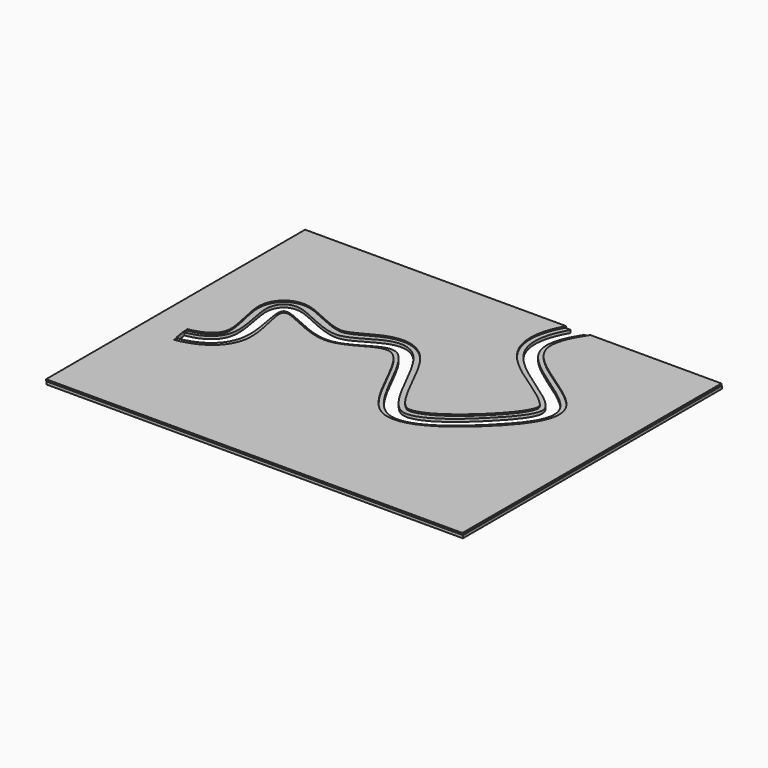
from build123d import *

# Parameters (mm, degrees)
F0_W          = 900
F0_H          = 700
F2_DEPTH      = 3
F3_DEPTH      = 25
F3_DEPTH_BACK = 25
F6_DEPTH      = 25
F6_DEPTH_BACK = 25
F7_W          = 900
F7_H          = 700
F9_DEPTH      = 6


# Not quite as in the source:
# - the dataset's text gives a spline's control points without its knots; the knots are read off the source's solid


with BuildPart() as f2:
    # F0 (on Top) → F2 (new body)
    with BuildSketch(Plane.XY):
        with Locations((136.779838565, 140.37967287)):
            Rectangle(F0_W, F0_H)
    extrude(amount=F2_DEPTH)

    # F1 (on Top) → F3 (cut, two sides)
    with BuildSketch(Plane.XY) as f3_sk:
        with BuildLine():
            Line((-241.4856788522, 82.2124957097), (-234.3062907457, 37.7888940275))
            add(Edge.make_bspline(
                [(-234.3062907457, 37.7888940275), (-183.2200698821, 46.0450414938), (-107.8197896412, 102.2279372719), (-192.2750551174, 283.579620296), (-24.0171318012, 149.9224145171), (99.4434854713, 307.8000943084), (175.8744786158, -38.137750164), (392.3120352571, 121.8215640239), (495.7588052716, 272.9639793915), (212.09229922, 380.1642280608), (301.8253737576, 491.1332534511), (345.4286754131, 545.0569987297)],
                knots=[0, 0, 0, 0, 0.1005186811, 0.1948714664, 0.2944457767, 0.3919205483, 0.524446972, 0.6500546131, 0.7560619639, 0.8852543369, 1, 1, 1, 1], degree=3))
            Line((345.4286754131, 545.0569987297), (310.4370311075, 573.3516064985))
            add(Edge.make_bspline(
                [(-241.4856788522, 82.2124957097), (-235.5376995244, 83.1737606775), (-227.1834080935, 85.1443072797), (-217.474364878, 88.6042185531), (-210.9663273096, 91.5416769635), (-205.2747075425, 94.7414795634), (-200.4160544418, 98.1187472011), (-196.373293023, 101.5953254918), (-193.0908775239, 105.1164927775), (-190.4790946185, 108.673215132), (-188.772395717, 111.7142206402), (-187.6443639611, 114.2600259837), (-186.91078749, 116.2492961693), (-186.2869465038, 118.3436017222), (-185.8604232074, 120.1988345417), (-185.5789375302, 121.7627021332), (-185.3991590865, 122.9783217928), (-185.252302169, 124.2414938638), (-185.1405994233, 125.5490498855), (-185.059563113, 126.9970714119), (-185.0000994287, 129.0879426638), (-185.0248632154, 131.9899533939), (-185.2286698235, 135.8675595467), (-185.6086882806, 140.0794825573), (-186.1581698074, 144.5682595729), (-187.0987121971, 150.8533570489), (-188.6205679067, 159.1522141918), (-190.8240279465, 169.5043124094), (-192.8083784067, 178.2695336381), (-194.3818406654, 185.3095616522), (-195.5285456157, 190.6070149505), (-196.6143456264, 195.9387036323), (-197.6084875244, 201.3452092887), (-198.4727294543, 206.9018156809), (-199.1496740668, 212.7389962035), (-199.4764712019, 218.0162233827), (-199.4894720296, 222.6632212336), (-199.3258979633, 226.4234804566), (-198.919614654, 230.5290516319), (-198.1659289654, 235.0572516522), (-196.9118918995, 240.0783575162), (-194.9451306123, 245.6253274688), (-192.4879995558, 250.6392221678), (-189.898614037, 254.7703034363), (-187.6218228143, 257.8777610524), (-184.9992992364, 260.934338153), (-182.0377655849, 263.8704376875), (-179.3129029064, 266.1548327791), (-177.000331504, 267.8542399638), (-174.6237907367, 269.4492377395), (-171.6062006951, 271.2068826251), (-167.9761634622, 272.9460428746), (-164.409661789, 274.3311498765), (-159.8065692755, 275.749902793), (-154.4349269126, 276.8203829827), (-148.7149350442, 277.3109893938), (-143.6791934777, 277.2781780434), (-139.2282351443, 276.9098327801), (-135.2505889333, 276.3274056454), (-131.6452560188, 275.6060761092), (-128.327829438, 274.7915830848), (-124.1994201874, 273.6177648935), (-119.454378243, 272.0297965106), (-114.1330202601, 269.9985841874), (-109.0163936944, 267.8708559657), (-104.0042481448, 265.6683344255), (-99.0398525291, 263.4119036969), (-94.0934068391, 261.1245526128), (-87.5071738324, 258.0675515109), (-79.2894636179, 254.301217329), (-69.5603592504, 250.1084557216), (-61.7384184503, 247.0939974118), (-55.7995425295, 245.0842808334), (-51.5499774528, 243.8013204219), (-47.5536122712, 242.7614646682), (-43.8633351999, 241.9756441117), (-41.0890345702, 241.5330763696), (-39.0767461943, 241.2996839349), (-37.6771518248, 241.1816399507), (-36.3922517161, 241.116479596), (-35.4214542607, 241.1018193712), (-34.7043651988, 241.1108325263), (-34.2011207672, 241.1268350515), (-33.6853437819, 241.1532206705), (-32.9848262391, 241.2026104861), (-32.080215541, 241.2918119898), (-30.9425191435, 241.4457711216), (-29.747492374, 241.6498724502), (-28.0732155104, 241.9930222828), (-25.822720168, 242.5627626208), (-21.880330047, 243.7981397699), (-16.331982542, 245.9761062402), (-8.8118359212, 249.5607949136), (-0.5434559099, 253.9526763782), (8.4508129905, 258.9262639267), (16.6403545663, 263.3417972682), (23.7599841554, 266.8841366803), (29.4467345634, 269.4962211057), (35.5566372376, 272.0010306462), (42.1823374373, 274.311405811), (49.4236395705, 276.3023826176), (57.3672041666, 277.795696083), (66.0465099256, 278.5509411968), (75.3837631228, 278.2821676865), (83.5113265637, 276.9778692101), (89.2081655274, 275.4330144664), (92.4367063904, 274.3708027239), (94.8382851466, 273.4852798104), (96.8161375588, 272.6754654295), (98.3841938016, 271.9843530185), (99.9262943401, 271.2721286966), (101.8038878917, 270.3453559302), (104.702705147, 268.7934917732), (108.1317869173, 266.7405344791), (111.9541425106, 264.1395026786), (115.5087239258, 261.4346763787), (119.927069824, 257.7228957042), (124.9169432693, 252.9328275462), (130.2508034542, 247.026543135), (135.0896327978, 240.9927455699), (139.554556696, 234.8416200953), (145.1283850319, 226.4875741975), (151.5589218926, 215.7632245239), (158.7710272688, 202.497891756), (165.6801971146, 188.9538806141), (172.4151365402, 175.2994869993), (179.0582911899, 161.7422451206), (185.660525585, 148.5206349377), (192.2444338178, 135.8994918833), (198.8008182512, 124.1678836236), (205.2768380346, 113.6369815809), (210.5101981, 106.1358052224), (214.4899104198, 101.0609993718), (217.3303617383, 97.7534217065), (219.978464374, 94.9733838681), (222.3765020584, 92.7378899598), (224.1137016073, 91.3274700325), (225.3142899389, 90.4567825785), (226.1163341361, 89.924057213), (226.8029845386, 89.5091405515), (227.4733439715, 89.1430138534), (228.1291176651, 88.822150909), (228.9996846256, 88.4432304879), (230.1054945245, 88.0467609434), (231.54537094, 87.6664964427), (233.1753732843, 87.3794091452), (235.057273097, 87.2021281247), (237.2335796296, 87.1635396823), (240.55731177, 87.3413929062), (245.5227987888, 88.079008451), (252.6791739242, 89.9923664451), (260.8301872351, 93.0264381942), (269.7570797741, 97.1825815618), (279.2556215065, 102.4009159936), (289.1468102787, 108.584934908), (299.2760739512, 115.6176345184), (309.5093899796, 123.3712014191), (319.7287874812, 131.7124258746), (329.8286859902, 140.5058445218), (338.0648038503, 148.0964177817), (344.5013770548, 154.2589683131), (348.4500767297, 158.1321041895), (351.5636214838, 161.2392515861), (354.6286384304, 164.3330415235), (358.3546871655, 168.163507658), (362.6480774345, 172.6981225537), (368.1173165148, 178.6510472941), (374.4439024175, 185.8985119346), (381.1201011492, 194.2088317575), (386.7882817119, 202.0338405705), (391.3723846707, 209.2487053252), (394.8283570488, 215.7004013288), (397.1689795838, 221.2164346332), (398.274140703, 224.8961691748), (398.7586304729, 227.2523477751), (398.9589780282, 228.7346603805), (399.033607176, 229.9543070221), (399.0177225056, 230.952451348), (398.9374713249, 231.7885688151), (398.8035372952, 232.5375385066), (398.6059933192, 233.282855915), (398.3615456687, 233.9702274749), (398.0917291127, 234.596295897), (397.885446547, 235.0253148368), (397.6933380765, 235.3947640399), (397.5351601954, 235.6845823574), (397.3594254936, 235.9919532357), (397.0874783947, 236.4470374628), (396.679784191, 237.0891477727), (395.8733663132, 238.2656919148), (394.567493912, 239.9926785021), (392.5131211223, 242.4074256407), (389.137265676, 246.0021498199), (383.7741089396, 251.0640022626), (375.751488869, 257.7405013236), (366.417496646, 264.8362812315), (356.0404038889, 272.2467658517), (344.8731898776, 279.9209527707), (333.1509121216, 287.8448474083), (321.0910339513, 296.0335168672), (308.893794176, 304.5289467569), (296.7425913103, 313.4033633299), (284.8049272706, 322.7684284522), (273.237915057, 332.7926592747), (264.0409228143, 341.9040126463), (257.0563649981, 349.8326975335), (252.0449681123, 356.1585682546), (248.1020472958, 361.7995109897), (245.1253394442, 366.5665889108), (242.9935925432, 370.2770521418), (241.3129881952, 373.4859400827), (240.0325980452, 376.1290050305), (238.8113517142, 378.7924683854), (237.3946194858, 382.1615894078), (235.3686208631, 387.6220814248), (233.2949562773, 394.552809555), (231.546773022, 402.9453959487), (230.5193972595, 411.3225036077), (230.1719914596, 419.6044271535), (230.4480888242, 427.7291455333), (231.5621988176, 438.2982923287), (234.1862414869, 450.9526422368), (238.8303853448, 465.2427656184), (244.6130062197, 478.7677873011), (251.2809191489, 491.6831883403), (258.6500420567, 504.1296805595), (266.5761934981, 516.2184522105), (274.935846315, 528.0312592745), (283.6149215817, 539.6249662726), (295.464949001, 554.8390039644), (304.4995700078, 566.0088107058), (310.4370311075, 573.3516064985)],
                knots=[0, 0, 0, 0, 0.015625, 0.0234375, 0.03125, 0.0390625, 0.046875, 0.0546875, 0.0625, 0.0703125, 0.078125, 0.08203125, 0.0859375, 0.08984375, 0.09375, 0.095703125, 0.09765625, 0.099609375, 0.1015625, 0.103515625, 0.10546875, 0.109375, 0.11328125, 0.1171875, 0.12109375, 0.125, 0.1328125, 0.140625, 0.1484375, 0.15234375, 0.15625, 0.16015625, 0.1640625, 0.16796875, 0.171875, 0.17578125, 0.177734375, 0.1796875, 0.181640625, 0.18359375, 0.185546875, 0.1875, 0.189453125, 0.1904296875, 0.19140625, 0.1923828125, 0.193359375, 0.1943359375, 0.1948242188, 0.1953125, 0.1962890625, 0.197265625, 0.1982421875, 0.19921875, 0.201171875, 0.203125, 0.205078125, 0.20703125, 0.208984375, 0.2109375, 0.212890625, 0.21484375, 0.21875, 0.22265625, 0.2265625, 0.23046875, 0.234375, 0.23828125, 0.2421875, 0.25, 0.2578125, 0.265625, 0.26953125, 0.2734375, 0.27734375, 0.28125, 0.28515625, 0.287109375, 0.2890625, 0.291015625, 0.29296875, 0.2939453125, 0.294921875, 0.2958984375, 0.296875, 0.298828125, 0.30078125, 0.302734375, 0.3046875, 0.30859375, 0.3125, 0.3203125, 0.328125, 0.3359375, 0.34375, 0.3515625, 0.35546875, 0.359375, 0.36328125, 0.3671875, 0.37109375, 0.375, 0.37890625, 0.3828125, 0.38671875, 0.388671875, 0.3896484375, 0.390625, 0.3916015625, 0.3920898438, 0.392578125, 0.3935546875, 0.39453125, 0.396484375, 0.3984375, 0.400390625, 0.40234375, 0.40625, 0.41015625, 0.4140625, 0.41796875, 0.421875, 0.4296875, 0.4375, 0.4453125, 0.453125, 0.4609375, 0.46875, 0.4765625, 0.484375, 0.4921875, 0.5, 0.50390625, 0.5078125, 0.51171875, 0.515625, 0.51953125, 0.521484375, 0.5234375, 0.525390625, 0.52734375, 0.529296875, 0.53125, 0.53515625, 0.5390625, 0.54296875, 0.546875, 0.55078125, 0.5546875, 0.5625, 0.5703125, 0.578125, 0.5859375, 0.59375, 0.6015625, 0.609375, 0.6171875, 0.625, 0.6328125, 0.640625, 0.64453125, 0.6484375, 0.650390625, 0.65234375, 0.65625, 0.66015625, 0.6640625, 0.671875, 0.6796875, 0.6875, 0.6953125, 0.703125, 0.7109375, 0.71875, 0.72265625, 0.7265625, 0.73046875, 0.734375, 0.73828125, 0.7421875, 0.74609375, 0.75, 0.751953125, 0.75390625, 0.7548828125, 0.755859375, 0.7568359375, 0.7578125, 0.759765625, 0.76171875, 0.765625, 0.76953125, 0.7734375, 0.78125, 0.7890625, 0.796875, 0.8046875, 0.8125, 0.8203125, 0.828125, 0.8359375, 0.84375, 0.8515625, 0.859375, 0.8671875, 0.87109375, 0.875, 0.87890625, 0.880859375, 0.8828125, 0.884765625, 0.8857421875, 0.88671875, 0.888671875, 0.890625, 0.89453125, 0.8984375, 0.90234375, 0.90625, 0.91015625, 0.9140625, 0.921875, 0.9296875, 0.9375, 0.9453125, 0.953125, 0.9609375, 0.96875, 0.9765625, 0.984375, 1, 1, 1, 1], degree=3))
        make_face()
    extrude(amount=F3_DEPTH, mode=Mode.SUBTRACT)
    extrude(f3_sk.sketch, amount=-F3_DEPTH_BACK, mode=Mode.SUBTRACT)


with BuildPart() as f2_1:
    # F5: moved
    add(f2.part.moved(Location((-139, -139, 6))))


with BuildPart() as f6:
    # F4 (on Top) → F6 (new body, two sides)
    with BuildSketch(Plane.XY) as f6_sk:
        with BuildLine():
            Line((-333.2689129169, -208.5999996712), (-329.2803639689, -233.2797783835))
            add(Edge.make_bspline(
                [(-329.2803639689, -233.2797783835), (-279.6440862088, -225.2579591544), (-215.0591975226, -169.0019007955), (-290.3221170229, 10.7279443108), (-115.933229477, -128.5278182105), (8.6171027688, 40.169951089), (91.4360122328, -317.6582258257), (294.4798541771, -146.0859910696), (390.4461045585, -16.0719332642), (105.2391975094, 95.5185231878), (204.8334747082, 217.5691570301), (250.45460219, 273.9883263187)],
                knots=[0, 0, 0, 0, 0.0976657324, 0.1914809372, 0.2938646504, 0.3927571199, 0.5271537272, 0.6507806642, 0.749994953, 0.8799442629, 1, 1, 1, 1], degree=3))
            Line((250.45460219, 273.9883263187), (231.014799798, 289.707552857))
            add(Edge.make_bspline(
                [(-333.2689129169, -208.5999996712), (-326.5356582324, -207.5118247648), (-317.1931037284, -205.2387950425), (-306.3838909726, -201.131018164), (-299.1159354338, -197.5685255044), (-292.6875905846, -193.5780513816), (-287.0795024379, -189.2040888935), (-282.2539728874, -184.4715031927), (-278.1616343726, -179.3755889151), (-274.7548284297, -173.8762725729), (-272.004457018, -167.9012394607), (-270.2621207217, -162.4489840488), (-269.3492323658, -158.3439603506), (-268.9196013639, -155.9107657182), (-268.6445813298, -154.0412952716), (-268.4179617417, -152.1250200421), (-268.2708607574, -150.4920692989), (-268.178315106, -149.1553098982), (-268.1017791313, -147.787649081), (-268.0366959253, -146.0273373624), (-268.0074636443, -143.83809812), (-268.0330013502, -140.8251744651), (-268.1836815232, -136.8974040515), (-268.5425410407, -131.9712532313), (-269.2358295256, -125.1762280136), (-270.4560911543, -116.3586946136), (-272.3017603747, -105.545902828), (-274.3259989971, -94.7403069697), (-276.3185069389, -84.1277531076), (-277.772685312, -75.5387465003), (-278.6910565664, -68.799797955), (-279.2187644678, -63.7788161512), (-279.5350356557, -58.733830778), (-279.5604611746, -53.5647284485), (-279.2250415257, -49.0206940891), (-278.6023825049, -45.1323212194), (-277.8982640923, -42.0603377083), (-276.8797273076, -38.8121645014), (-275.4455548583, -35.3892511345), (-273.4790588951, -31.8374466759), (-271.305823316, -28.8665182353), (-269.2236062579, -26.5816714906), (-267.4957329052, -24.9446019313), (-265.9272233847, -23.6693040063), (-264.6061679224, -22.7168534474), (-263.5845965554, -22.0387788556), (-262.5400095899, -21.4024713172), (-261.1379217102, -20.6202936087), (-259.3723656238, -19.7624478141), (-257.2664768815, -18.9191927957), (-254.5077179753, -18.0245960695), (-251.2000220802, -17.2947134288), (-247.526764406, -16.8905642308), (-244.1461911465, -16.8266916994), (-241.0218040198, -17.0055225982), (-238.1058387703, -17.3595544011), (-234.4344132952, -18.0062082748), (-230.1461571265, -19.0650837496), (-225.2401991321, -20.6081155776), (-220.428560194, -22.3650098202), (-215.6241958309, -24.2977102764), (-209.1635726945, -27.0686912343), (-200.91533098, -30.8248650185), (-190.6992823023, -35.5633740418), (-180.2474658182, -40.2795972838), (-169.7035594185, -44.7101422758), (-159.2590572075, -48.5915934212), (-150.833086294, -51.1595912285), (-144.3969270885, -52.708623803), (-139.7597894843, -53.5984287402), (-135.350217645, -54.2021923049), (-131.8947581809, -54.4618466023), (-129.2773886965, -54.5250055118), (-127.3886195937, -54.5012672263), (-125.5834761423, -54.4084821332), (-123.75735039, -54.2430127225), (-121.9179256246, -54.0060449492), (-119.4386939412, -53.5950915733), (-115.0236778915, -52.6281983161), (-108.464450337, -50.5461688208), (-100.209458435, -47.0145503997), (-91.6473177788, -42.6292695447), (-82.8356633205, -37.6323659906), (-73.7820326342, -32.2980788941), (-64.4204788343, -26.9162564968), (-56.2244895109, -22.6463808947), (-49.2756699808, -19.5487355759), (-43.8133941483, -17.4497347779), (-38.0428319595, -15.6577145741), (-31.9100593387, -14.2848925391), (-25.3863705909, -13.4787706401), (-18.5000233839, -13.4165023579), (-12.557265223, -14.133129136), (-7.7865894592, -15.2265427799), (-4.8246097736, -16.1301935238), (-2.4830188095, -16.984188282), (-0.7427660824, -17.6899007664), (0.9709845891, -18.4568454065), (3.1885919534, -19.5421936723), (5.8485426274, -21.0115303516), (9.8718071452, -23.5627825113), (14.5000714326, -27.0687833334), (19.5365876981, -31.6576976572), (24.1739882822, -36.5623991895), (28.5076750141, -41.7464765079), (32.6112471084, -47.1880102691), (37.8488651353, -54.764030926), (44.0654277581, -64.7959256173), (51.2201351181, -77.5865758044), (58.2026287306, -90.9485676633), (65.1030299231, -104.6722368616), (71.9847087497, -118.5258924104), (78.8933104853, -132.2605289934), (85.8592210003, -145.6123778219), (92.8961025164, -158.3039513189), (99.9953000632, -170.0442708674), (107.1143439792, -180.530730928), (112.9853173881, -187.9673444171), (117.5571297552, -192.9928132518), (120.891347435, -196.2718180315), (123.5607943849, -198.5789440356), (125.6110125922, -200.1666005585), (127.1013954479, -201.2296275031), (128.299871881, -202.0106634877), (129.2319913269, -202.5751821399), (130.1420372188, -203.0981419586), (131.2710187578, -203.6944665479), (132.626458923, -204.3302155974), (133.9864461835, -204.8908623689), (135.8156146818, -205.545292611), (138.1487884217, -206.198760127), (141.077635188, -206.7370218737), (145.2141858408, -207.1274073481), (150.9064499461, -206.9767427556), (158.6590034827, -205.6449354418), (167.244272616, -203.074417377), (176.5043495372, -199.2617251909), (186.269555269, -194.2698704354), (196.3839518787, -188.2045424102), (206.7110295818, -181.1952498955), (217.1322533607, -173.3837647463), (227.5435683457, -164.9175624249), (237.8519285523, -155.9463690586), (247.9727234425, -146.6201938313), (256.1846315059, -138.6774946859), (262.5848873219, -132.2944036856), (267.2896553578, -127.5126499147), (271.8985046876, -122.748219897), (276.3517380743, -118.064097177), (280.6360934064, -113.4597602), (286.1050318739, -107.4319261502), (292.4503775362, -100.1139582853), (299.1710967524, -91.7191679074), (304.8952626236, -83.7698370339), (309.5342332929, -76.3475286822), (313.0297660901, -69.5576730595), (315.3796022741, -63.5166343333), (316.4534174009, -59.1803878595), (316.8684624481, -56.1104390775), (316.9825551901, -53.9805609293), (316.9189582881, -51.9841685855), (316.6870514368, -50.0672519618), (316.2805485965, -48.1671369792), (315.7761402691, -46.5443817923), (315.2528137353, -45.1946320684), (314.7940046118, -44.150856615), (314.3510194684, -43.2510672458), (313.9563962067, -42.5107950014), (313.6403277182, -41.946580014), (313.2996180656, -41.3666861232), (312.8071634118, -40.5653642298), (312.1212354569, -39.5166101946), (311.1830626083, -38.1877669006), (309.7784964594, -36.3308443648), (307.7357978991, -33.8650208604), (304.8404403301, -30.7178973681), (301.5251654901, -27.4183194333), (296.5833748239, -22.8530326503), (289.5064042219, -16.8926708352), (279.8319575373, -9.4512466565), (269.227680549, -1.7805411734), (257.934312506, 6.0926856509), (246.1812875466, 14.1644513549), (234.1876053412, 22.4474173419), (222.1627658357, 30.9689201568), (210.3075244762, 39.7718879334), (198.8148664416, 48.9186823586), (187.8729843469, 58.4986195172), (179.3718553715, 66.9485512729), (173.0482225424, 74.0787256506), (168.5766093857, 79.6400266203), (164.4138513635, 85.4456908838), (161.2410767319, 90.514082676), (158.9095794021, 94.7226214256), (157.2734640868, 97.9573725172), (155.75735069, 101.2794930253), (154.3903989976, 104.6366271066), (153.1706645122, 108.0265936891), (151.7416942377, 112.581548034), (149.756114357, 120.6251220695), (148.3634532991, 132.2007283871), (148.7712889539, 145.9093868829), (150.9390302606, 159.2673485535), (154.5610013717, 172.2378616731), (159.3830697519, 184.856918191), (165.2034437031, 197.1847219475), (171.8581554162, 209.2797407613), (181.656654805, 225.1567879701), (195.3201464248, 244.6214659901), (213.0280067843, 267.48337337), (225.0836440416, 282.3725548162), (231.014799798, 289.707552857)],
                knots=[0, 0, 0, 0, 0.015625, 0.0234375, 0.03125, 0.0390625, 0.046875, 0.0546875, 0.0625, 0.0703125, 0.078125, 0.0859375, 0.08984375, 0.091796875, 0.09375, 0.095703125, 0.09765625, 0.0986328125, 0.099609375, 0.1015625, 0.103515625, 0.10546875, 0.109375, 0.11328125, 0.1171875, 0.125, 0.1328125, 0.140625, 0.1484375, 0.15625, 0.16015625, 0.1640625, 0.16796875, 0.171875, 0.17578125, 0.177734375, 0.1796875, 0.181640625, 0.18359375, 0.185546875, 0.1875, 0.1884765625, 0.189453125, 0.1904296875, 0.1909179688, 0.19140625, 0.1918945312, 0.1923828125, 0.193359375, 0.1943359375, 0.1953125, 0.197265625, 0.19921875, 0.201171875, 0.203125, 0.205078125, 0.20703125, 0.2109375, 0.21484375, 0.21875, 0.22265625, 0.2265625, 0.234375, 0.2421875, 0.25, 0.2578125, 0.265625, 0.2734375, 0.27734375, 0.28125, 0.28515625, 0.2890625, 0.291015625, 0.29296875, 0.294921875, 0.296875, 0.298828125, 0.30078125, 0.3046875, 0.3125, 0.3203125, 0.328125, 0.3359375, 0.34375, 0.3515625, 0.359375, 0.36328125, 0.3671875, 0.37109375, 0.375, 0.37890625, 0.3828125, 0.38671875, 0.388671875, 0.390625, 0.3916015625, 0.392578125, 0.3935546875, 0.39453125, 0.396484375, 0.3984375, 0.40234375, 0.40625, 0.41015625, 0.4140625, 0.41796875, 0.421875, 0.4296875, 0.4375, 0.4453125, 0.453125, 0.4609375, 0.46875, 0.4765625, 0.484375, 0.4921875, 0.5, 0.5078125, 0.51171875, 0.515625, 0.51953125, 0.521484375, 0.5234375, 0.525390625, 0.5263671875, 0.52734375, 0.529296875, 0.53125, 0.533203125, 0.53515625, 0.5390625, 0.54296875, 0.546875, 0.5546875, 0.5625, 0.5703125, 0.578125, 0.5859375, 0.59375, 0.6015625, 0.609375, 0.6171875, 0.625, 0.6328125, 0.640625, 0.64453125, 0.6484375, 0.65234375, 0.65625, 0.66015625, 0.6640625, 0.671875, 0.6796875, 0.6875, 0.6953125, 0.703125, 0.7109375, 0.71875, 0.72265625, 0.7265625, 0.73046875, 0.734375, 0.73828125, 0.7421875, 0.744140625, 0.74609375, 0.748046875, 0.7490234375, 0.75, 0.7509765625, 0.751953125, 0.75390625, 0.755859375, 0.7578125, 0.76171875, 0.765625, 0.76953125, 0.7734375, 0.78125, 0.7890625, 0.796875, 0.8046875, 0.8125, 0.8203125, 0.828125, 0.8359375, 0.84375, 0.8515625, 0.859375, 0.86328125, 0.8671875, 0.87109375, 0.875, 0.876953125, 0.87890625, 0.880859375, 0.8828125, 0.884765625, 0.88671875, 0.890625, 0.8984375, 0.90625, 0.9140625, 0.921875, 0.9296875, 0.9375, 0.9453125, 0.953125, 0.96875, 0.984375, 1, 1, 1, 1], degree=3))
        make_face()
    extrude(amount=F6_DEPTH)
    extrude(f6_sk.sketch, amount=-F6_DEPTH_BACK)


with BuildPart() as f6_1:
    # F8: moved
    add(f6.part.moved(Location((-47, 144, 0))))


with BuildPart() as f9:
    # F7 (on Top) → F9 (new body)
    with BuildSketch(Plane.XY):
        Rectangle(F7_W, F7_H)
    extrude(amount=F9_DEPTH)

    # F10: cut F6
    add(f6_1.part, mode=Mode.SUBTRACT)


with BuildPart() as f2_2:
    add(f2_1.part)

    # F10: cut F6
    add(f6_1.part, mode=Mode.SUBTRACT)


solid = Compound([f9.part, f2_2.part])
